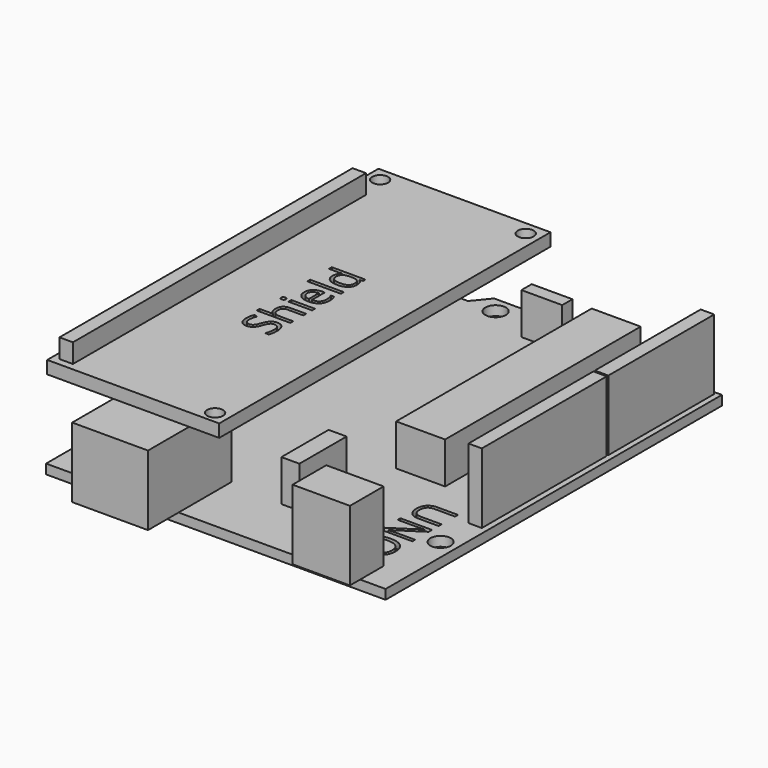
from build123d import *

# Parameters (mm, degrees)
F0_R          = 1.608
F0_W          = 2.0698662847
F0_H          = 16.1716472358
F0_W_2        = 2.8245758731
F0_H_2        = 9.258328937
F0_W_3        = 2.0288862288
F0_H_3        = 29.093706049
F0_W_4        = 7.6891221106
F0_H_4        = 38.3777157404
F0_W_5        = 2.0933430642
F0_H_5        = 24.5057968423
F0_W_6        = 6.3997777761
F0_H_6        = 2.006649971
F0_W_7        = 2.1252632141
F0_H_7        = 20.775090903
F0_TEXT_SIZE  = 6.9444444444
F1_DEPTH      = 1.5
F0_W_8        = 11.9
F0_H_8        = 6
F0_H_9        = 10.374043391
F0_W_9        = 9
F0_H_10       = 4.6058264838
F0_H_11       = 2
F2_DEPTH      = 12.5
F3_DEPTH      = 8
F5_W          = 27
F5_H          = 65
F5_W_2        = 2.1082367748
F5_H_2        = 57.5133208185
F5_R          = 1.25
F6_DEPTH      = 2
F7_DEPTH      = 5
F9_TEXT_SIZE  = 6.9444444444
F10_DEPTH     = 1
F11_TEXT_SIZE = 6.9444444444
F12_DEPTH     = 1
F13_DEPTH     = 1.5


# Not quite as in the source:
# - a feature names something its author has since deleted; it is built from what else it names
# - Text() gives the source's letters only with a copy of the font that has no kerning and outlines rounded to 1/6400 em; it was checked with that copy


with BuildPart() as f1:
    # F0 (on Top) → F1 (new body)
    with BuildSketch(Plane.XY):
        with BuildLine():
            Line((26.65, -32.99775), (26.65, 32.99775))
            Line((26.65, 32.99775), (23.0735316873, 32.99775))
            Line((23.0735316873, 32.99775), (20.6407, 32.99775))
            ThreePointArc((20.6407, 32.99775), (19.0327, 31.38975), (17.4247, 32.99775))
            Line((17.4247, 32.99775), (-7.2683, 32.99775))
            ThreePointArc((-7.2683, 32.99775), (-8.8763, 31.38975), (-10.4843, 32.99775))
            Line((-10.4843, 32.99775), (-13.2244247943, 32.99775))
            Line((-13.2244247943, 32.99775), (-26.65, 32.99775))
            Line((-26.65, 32.99775), (-26.65, -32.99775))
            Line((-26.65, -32.99775), (-17.75, -32.99775))
            Line((-17.75, -32.99775), (-17.75, -22.623706609))
            Line((-17.75, -22.623706609), (-5.85, -22.623706609))
            Line((-5.85, -22.623706609), (-5.85, -32.99775))
            Line((-5.85, -32.99775), (13.65, -32.99775))
            Line((13.65, -32.99775), (13.65, -28.3919235162))
            Line((13.65, -28.3919235162), (22.65, -28.3919235162))
            Line((22.65, -28.3919235162), (22.65, -32.99775))
            Line((22.65, -32.99775), (26.65, -32.99775))
        make_face()
        with Locations((-24.1109, -17.76315)):
            Circle(F0_R, mode=Mode.SUBTRACT)
        with Locations((-24.858337827, -4.9088280648)):
            Rectangle(F0_W, F0_H, mode=Mode.SUBTRACT)
        with BuildLine():
            add(Edge.make_bspline(
                [(19.0838481378, -24.1438748605), (18.405679735, -24.7439182632), (17.2121033461, -24.7439182632)],
                knots=[0, 0, 0, 1, 1, 1], degree=2))
            add(Edge.make_bspline(
                [(17.2121033461, -24.7439182632), (16.0217821655, -24.7439182632), (15.3398160197, -24.1417047216)],
                knots=[0, 0, 0, 1, 1, 1], degree=2))
            add(Edge.make_bspline(
                [(15.3398160197, -24.1417047216), (14.6578498739, -23.5394911799), (14.6578498739, -22.4685276382)],
                knots=[0, 0, 0, 1, 1, 1], degree=2))
            add(Edge.make_bspline(
                [(14.6578498739, -22.4685276382), (14.6578498739, -21.3736925688), (15.3278802558, -20.7785319785)],
                knots=[0, 0, 0, 1, 1, 1], degree=2))
            add(Edge.make_bspline(
                [(15.3278802558, -20.7785319785), (15.9979106378, -20.1833713882), (17.2186137628, -20.1833713882)],
                knots=[0, 0, 0, 1, 1, 1], degree=2))
            add(Edge.make_bspline(
                [(17.2186137628, -20.1833713882), (18.4295512628, -20.1833713882), (19.0957839016, -20.7801595827)],
                knots=[0, 0, 0, 1, 1, 1], degree=2))
            add(Edge.make_bspline(
                [(19.0957839016, -20.7801595827), (19.7620165405, -21.3769477771), (19.7620165405, -22.4750380549)],
                knots=[0, 0, 0, 1, 1, 1], degree=2))
            add(Edge.make_bspline(
                [(19.7620165405, -22.4750380549), (19.7620165405, -23.5438314577), (19.0838481378, -24.1438748605)],
                knots=[0, 0, 0, 1, 1, 1], degree=2))
        make_face(mode=Mode.SUBTRACT)
        with Locations((4.0160067147, -18.7563267536)):
            Rectangle(F0_W_2, F0_H_2, mode=Mode.SUBTRACT)
        with BuildLine():
            Line((19.6838915405, -19.0776856244), (14.7262092489, -19.0776856244))
            Line((14.7262092489, -19.0776856244), (14.7262092489, -18.420133541))
            Line((14.7262092489, -18.420133541), (18.8863654989, -15.7107151382))
            Line((18.8863654989, -15.7107151382), (18.8863654989, -15.6835884021))
            add(Edge.make_bspline(
                [(18.8863654989, -15.6835884021), (18.1539436239, -15.7378418744), (17.5441345961, -15.7378418744)],
                knots=[0, 0, 0, 1, 1, 1], degree=2))
            Line((17.5441345961, -15.7378418744), (14.7262092489, -15.7378418744))
            Line((14.7262092489, -15.7378418744), (14.7262092489, -15.2050727771))
            Line((14.7262092489, -15.2050727771), (19.6838915405, -15.2050727771))
            Line((19.6838915405, -15.2050727771), (19.6838915405, -15.8561144438))
            Line((19.6838915405, -15.8561144438), (15.5400113322, -18.5590224299))
            Line((15.5400113322, -18.5590224299), (15.5400113322, -18.586149166))
            add(Edge.make_bspline(
                [(15.5400113322, -18.586149166), (15.6311571655, -18.5796387494), (16.1281189711, -18.5557672216)],
                knots=[0, 0, 0, 1, 1, 1], degree=2))
            add(Edge.make_bspline(
                [(16.1281189711, -18.5557672216), (16.6250807766, -18.5318956938), (16.8388394572, -18.5384061105)],
                knots=[0, 0, 0, 1, 1, 1], degree=2))
            Line((16.8388394572, -18.5384061105), (19.6838915405, -18.5384061105))
            Line((19.6838915405, -18.5384061105), (19.6838915405, -19.0776856244))
        make_face(mode=Mode.SUBTRACT)
        with BuildLine():
            Line((19.6838915405, -13.3170519438), (19.6838915405, -13.8932238188))
            Line((19.6838915405, -13.8932238188), (16.4764262628, -13.8932238188))
            add(Edge.make_bspline(
                [(16.4764262628, -13.8932238188), (15.6279019572, -13.8932238188), (15.1428759155, -13.381071041)],
                knots=[0, 0, 0, 1, 1, 1], degree=2))
            add(Edge.make_bspline(
                [(15.1428759155, -13.381071041), (14.6578498739, -12.8689182632), (14.6578498739, -11.9737359716)],
                knots=[0, 0, 0, 1, 1, 1], degree=2))
            add(Edge.make_bspline(
                [(14.6578498739, -11.9737359716), (14.6578498739, -11.0785536799), (15.1466736586, -10.5886448257)],
                knots=[0, 0, 0, 1, 1, 1], degree=2))
            add(Edge.make_bspline(
                [(15.1466736586, -10.5886448257), (15.6354974433, -10.0987359716), (16.4894470961, -10.0987359716)],
                knots=[0, 0, 0, 1, 1, 1], degree=2))
            Line((16.4894470961, -10.0987359716), (19.6838915405, -10.0987359716))
            Line((19.6838915405, -10.0987359716), (19.6838915405, -10.675992916))
            Line((19.6838915405, -10.675992916), (16.4492995266, -10.675992916))
            add(Edge.make_bspline(
                [(16.4492995266, -10.675992916), (15.8286398044, -10.675992916), (15.4960660197, -11.0150771174)],
                knots=[0, 0, 0, 1, 1, 1], degree=2))
            add(Edge.make_bspline(
                [(15.4960660197, -11.0150771174), (15.163492235, -11.3541613188), (15.163492235, -12.0117134021)],
                knots=[0, 0, 0, 1, 1, 1], degree=2))
            add(Edge.make_bspline(
                [(15.163492235, -12.0117134021), (15.163492235, -12.638883541), (15.4976936239, -12.9779677424)],
                knots=[0, 0, 0, 1, 1, 1], degree=2))
            add(Edge.make_bspline(
                [(15.4976936239, -12.9779677424), (15.8318950128, -13.3170519438), (16.4558099433, -13.3170519438)],
                knots=[0, 0, 0, 1, 1, 1], degree=2))
            Line((16.4558099433, -13.3170519438), (19.6838915405, -13.3170519438))
        make_face(mode=Mode.SUBTRACT)
        with Locations((24.1109, -19.03265)):
            Circle(F0_R, mode=Mode.SUBTRACT)
        with Locations((-24.8669572175, 18.1186790578)):
            Rectangle(F0_W_3, F0_H_3, mode=Mode.SUBTRACT)
        with Locations((11.5096539375, 11.9860179257)):
            Rectangle(F0_W_4, F0_H_4, mode=Mode.SUBTRACT)
        with Locations((24.705122225, -0.7417532615)):
            Rectangle(F0_W_5, F0_H_5, mode=Mode.SUBTRACT)
        with Locations((1.0835805733, 30.6235402822)):
            Rectangle(F0_W_6, F0_H_6, mode=Mode.SUBTRACT)
        with Locations((24.7146608829, 22.1882332116)):
            Rectangle(F0_W_7, F0_H_7, mode=Mode.SUBTRACT)
        with BuildLine():
            Line((20.6407, 32.99775), (23.0735316873, 32.99775))
            Line((23.0735316873, 32.99775), (20.7428282746, 35.53685))
            Line((20.7428282746, 35.53685), (-11.145020587, 35.53685))
            Line((-11.145020587, 35.53685), (-13.2244247943, 32.99775))
            Line((-13.2244247943, 32.99775), (-10.4843, 32.99775))
            ThreePointArc((-10.4843, 32.99775), (-8.8763, 34.60575), (-7.2683, 32.99775))
            Line((-7.2683, 32.99775), (17.4247, 32.99775))
            ThreePointArc((17.4247, 32.99775), (19.0327, 34.60575), (20.6407, 32.99775))
        make_face()
        with BuildLine():
            add(Edge.make_bspline(
                [(18.7257752211, -21.2223253813), (18.2049418878, -20.793180416), (17.2121033461, -20.793180416)],
                knots=[0, 0, 0, 1, 1, 1], degree=2))
            add(Edge.make_bspline(
                [(17.2121033461, -20.793180416), (16.2051589016, -20.793180416), (15.6843255683, -21.2223253813)],
                knots=[0, 0, 0, 1, 1, 1], degree=2))
            add(Edge.make_bspline(
                [(15.6843255683, -21.2223253813), (15.163492235, -21.6514703466), (15.163492235, -22.4685276382)],
                knots=[0, 0, 0, 1, 1, 1], degree=2))
            add(Edge.make_bspline(
                [(15.163492235, -22.4685276382), (15.163492235, -23.2920953466), (15.6821554294, -23.7125597563)],
                knots=[0, 0, 0, 1, 1, 1], degree=2))
            add(Edge.make_bspline(
                [(15.6821554294, -23.7125597563), (16.2008186239, -24.133024166), (17.2121033461, -24.133024166)],
                knots=[0, 0, 0, 1, 1, 1], degree=2))
            add(Edge.make_bspline(
                [(17.2121033461, -24.133024166), (18.2125373739, -24.133024166), (18.7295729641, -23.7141873605)],
                knots=[0, 0, 0, 1, 1, 1], degree=2))
            add(Edge.make_bspline(
                [(18.7295729641, -23.7141873605), (19.2466085544, -23.2953505549), (19.2466085544, -22.4750380549)],
                knots=[0, 0, 0, 1, 1, 1], degree=2))
            add(Edge.make_bspline(
                [(19.2466085544, -22.4750380549), (19.2466085544, -21.6514703466), (18.7257752211, -21.2223253813)],
                knots=[0, 0, 0, 1, 1, 1], degree=2))
        make_face()
        with Locations(Location((14.7262092489, -9.4683106244), (0, 0, -90))):
            Text('UNO', F0_TEXT_SIZE, font='Open Sans', text_align=(TextAlign.LEFT, TextAlign.BOTTOM))
    extrude(amount=F1_DEPTH)

    # F0 (on Top) → F2 (join)
    with BuildSketch(Plane.XY):
        with Locations((-24.8669572175, 18.1186790578)):
            Rectangle(F0_W_3, F0_H_3)
        with Locations((24.7146608829, 22.1882332116)):
            Rectangle(F0_W_7, F0_H_7)
        with Locations((24.705122225, -0.7417532615)):
            Rectangle(F0_W_5, F0_H_5)
        with Locations((-24.858337827, -4.9088280648)):
            Rectangle(F0_W, F0_H)
        with Locations((-11.8, -35.99775)):
            Rectangle(F0_W_8, F0_H_8)
        with Locations((-11.8, -27.8107283045)):
            Rectangle(F0_W_8, F0_H_9)
        with Locations((18.15, -30.6948367581)):
            Rectangle(F0_W_9, F0_H_10)
        with Locations((18.15, -33.99775)):
            Rectangle(F0_W_9, F0_H_11)
    extrude(amount=F2_DEPTH)

    # F0 (on Top) → F3 (join)
    with BuildSketch(Plane.XY):
        with Locations((11.5096539375, 11.9860179257)):
            Rectangle(F0_W_4, F0_H_4)
        with Locations((1.0835805733, 30.6235402822)):
            Rectangle(F0_W_6, F0_H_6)
        with Locations((4.0160067147, -18.7563267536)):
            Rectangle(F0_W_2, F0_H_2)
    extrude(amount=F3_DEPTH)

    # F9 (on offset) → F10 (cut)
    with BuildSketch(Plane.XY.offset(1.5)):
        with Locations(Location((16.3420995506, -11.4649879932), (0, 0, -90))):
            Text('UNO', F9_TEXT_SIZE, font='Open Sans', text_align=(TextAlign.LEFT, TextAlign.BOTTOM))
    extrude(amount=-F10_DEPTH, mode=Mode.SUBTRACT)

    # F0 (on Top) → F13 (cut)
    with BuildSketch(Plane.XY):
        with Locations((18.15, -33.99775)):
            Rectangle(F0_W_9, F0_H_11)
        with Locations((-11.8, -35.99775)):
            Rectangle(F0_W_8, F0_H_8)
    extrude(amount=F13_DEPTH, mode=Mode.SUBTRACT)


with BuildPart() as f6:
    # F5 (on offset) → F6 (new body)
    with BuildSketch(Plane.XY.offset(12.5)):
        with Locations((-14.6296425541, 1.5757660754)):
            Rectangle(F5_W, F5_H)
        with Locations((-26.0432483628, -1.0521514341)):
            Rectangle(F5_W_2, F5_H_2, mode=Mode.SUBTRACT)
        with Locations((-3.280660836, -29.0467493153)):
            Circle(F5_R, mode=Mode.SUBTRACT)
        with Locations((-26.140660836, 31.9132506847)):
            Circle(F5_R, mode=Mode.SUBTRACT)
        with Locations((-3.280660836, 31.9132506847)):
            Circle(F5_R, mode=Mode.SUBTRACT)
    extrude(amount=F6_DEPTH)

    # F11 (on face) → F12 (cut)
    with BuildSketch(Plane.XY.offset(14.5)):
        with Locations(Location((-10.9837375664, -9.0497257888), (0, 0, 90))):
            Text('Shield', F11_TEXT_SIZE, font='Open Sans', text_align=(TextAlign.LEFT, TextAlign.BOTTOM))
    extrude(amount=-F12_DEPTH, mode=Mode.SUBTRACT)


with BuildPart() as f7:
    # F5 (on offset) → F7 (new body)
    with BuildSketch(Plane.XY.offset(12.5)):
        with Locations((-26.0432483628, -1.0521514341)):
            Rectangle(F5_W_2, F5_H_2)
    extrude(amount=F7_DEPTH)


solid = Compound([f1.part, f6.part, f7.part])
